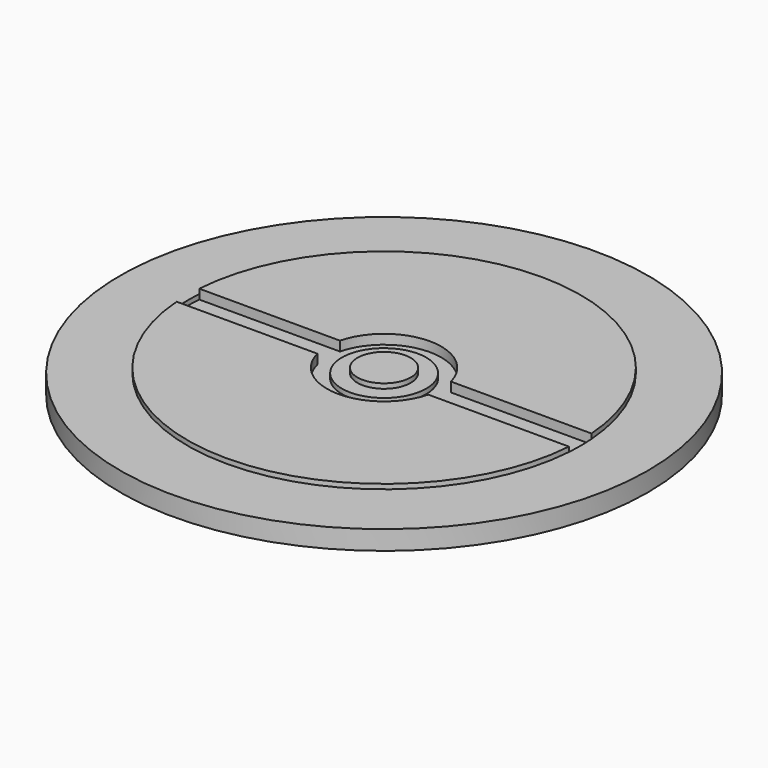
from build123d import *

# Parameters (mm, degrees)
F0_R      = 55.0458583504
F1_DEPTH  = 4
F2_R      = 41.0058886934
F3_DEPTH  = 1
F4_R      = 11.9318178019
F5_DEPTH  = 2
F6_R      = 8.7944266384
F7_DEPTH  = 1
F8_R      = 5.553220806
F9_DEPTH  = 1
F11_DEPTH = 2
F13_DEPTH = 2


with BuildPart() as f1:
    # F0 (on Top) → F1 (new body)
    with BuildSketch(Plane.XY):
        Circle(F0_R)
    extrude(amount=F1_DEPTH)

    # F2 (on face) → F3 (join)
    with BuildSketch(Plane.XY.offset(4)):
        Circle(F2_R)
    extrude(amount=F3_DEPTH)

    # F4 (on face) → F5 (cut)
    with BuildSketch(Plane.XY.offset(5)):
        Circle(F4_R)
    extrude(amount=-F5_DEPTH, mode=Mode.SUBTRACT)

    # F6 (on face) → F7 (join)
    with BuildSketch(Plane.XY.offset(3)):
        Circle(F6_R)
    extrude(amount=F7_DEPTH)

    # F8 (on face) → F9 (join)
    with BuildSketch(Plane.XY.offset(4)):
        Circle(F8_R)
    extrude(amount=F9_DEPTH)

    # F10 (on face) → F11 (cut)
    with BuildSketch(Plane.XY.offset(5)):
        with BuildLine():
            Line((-11.5631810567, 2.9429780682), (-40.9001441028, 2.9429780682))
            ThreePointArc((-40.9001441028, 2.9429780682), (-41.0058886934, 0), (-40.9001441028, -2.9429780682))
            Line((-40.9001441028, -2.9429780682), (-11.5631810567, -2.9429780682))
            ThreePointArc((-11.5631810567, -2.9429780682), (-11.9318178019, 0), (-11.5631810567, 2.9429780682))
        make_face()
    extrude(amount=-F11_DEPTH, mode=Mode.SUBTRACT)

    # F12 (on face) → F13 (cut)
    with BuildSketch(Plane.XY.offset(5)):
        with BuildLine():
            Line((40.8989598294, 2.959390547), (11.5589914633, 2.959390547))
            ThreePointArc((11.5589914633, 2.959390547), (11.9318147961, 0.0084693883), (11.5631810567, -2.9429780682))
            Line((11.5631810567, -2.9429780682), (40.9001441028, -2.9429780682))
            ThreePointArc((40.9001441028, -2.9429780682), (41.005887868, 0.008227575), (40.8989598294, 2.959390547))
        make_face()
    extrude(amount=-F13_DEPTH, mode=Mode.SUBTRACT)


solid = f1.part
